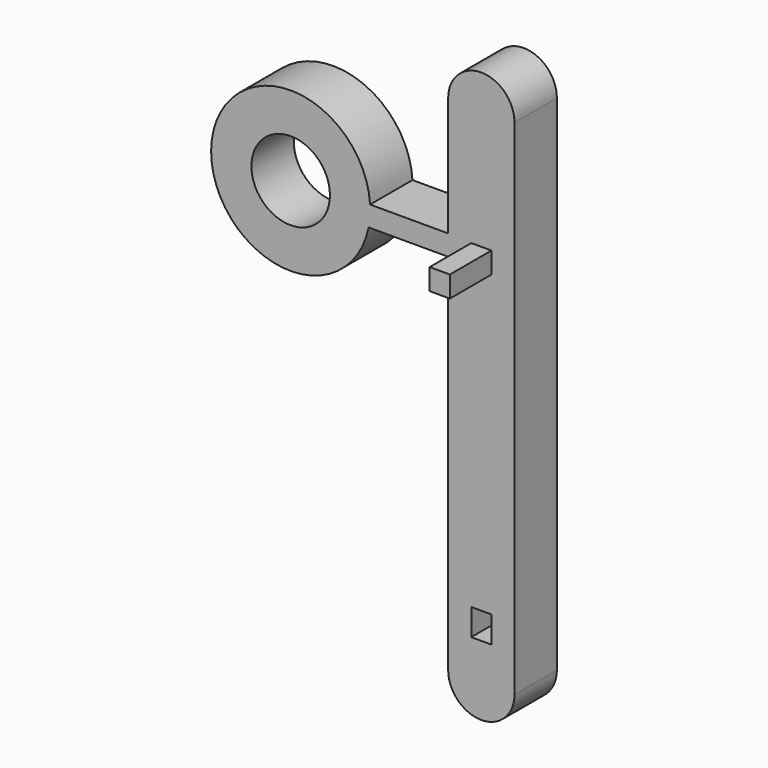
from build123d import *

# Parameters (mm, degrees)
F0_R     = 4.7018325436
F0_W     = 2.4090255611
F0_H     = 3.1813085079
F0_W_2   = 2.413
F0_H_2   = 2.54
F1_DEPTH = 3.175
F2_DEPTH = 9.398
F3_DEPTH = 3.175


# Not quite as in the source:
# - a feature names something its author has since deleted; it is built from what else it names


with BuildPart() as f1:
    # F0 (on Front) → F1 (new body, symmetric)
    with BuildSketch(Plane.XZ):
        with BuildLine():
            ThreePointArc((-13.3044686056, 15.3006398952), (-13.3088027932, 15.5879506834), (-13.3218014117, 15.875))
            ThreePointArc((-13.3218014117, 15.875), (-32.3313565604, 15.9637766028), (-13.49375, 13.4112))
            ThreePointArc((-13.49375, 13.4112), (-13.3519070859, 14.3511912968), (-13.3044686056, 15.3006398952))
        make_face()
        with Locations((-22.8294686056, 15.3006398952)):
            Circle(F0_R, mode=Mode.SUBTRACT)
        with BuildLine():
            Line((-3.96875, 13.4112), (-3.96875, 15.875))
            Line((-3.96875, 15.875), (-13.3218014117, 15.875))
            ThreePointArc((-13.3218014117, 15.875), (-13.3088027932, 15.5879506834), (-13.3044686056, 15.3006398952))
            ThreePointArc((-13.3044686056, 15.3006398952), (-13.3519070859, 14.3511912968), (-13.49375, 13.4112))
            Line((-13.49375, 13.4112), (-3.96875, 13.4112))
        make_face()
        with BuildLine():
            Line((3.96875, -30.1625), (3.96875, 30.1625))
            ThreePointArc((3.96875, 30.1625), (0, 34.13125), (-3.96875, 30.1625))
            Line((-3.96875, 30.1625), (-3.96875, 15.875))
            Line((-3.96875, 15.875), (-3.96875, 13.4112))
            Line((-3.96875, 13.4112), (-3.96875, -30.1625))
            ThreePointArc((-3.96875, -30.1625), (0, -34.13125), (3.96875, -30.1625))
        make_face()
        with Locations((0, -24.1956412792)):
            Rectangle(F0_W, F0_H, mode=Mode.SUBTRACT)
        with Locations((0, 14.4846439362)):
            Rectangle(F0_W_2, F0_H_2, mode=Mode.SUBTRACT)
    extrude(amount=F1_DEPTH, both=True)

    # F0 (on Front) → F2 (join)
    with BuildSketch(Plane.XZ):
        with Locations((0, 14.4846439362)):
            Rectangle(F0_W_2, F0_H_2)
    extrude(amount=F2_DEPTH)

    # F0 (on Front) → F3 (join)
    with BuildSketch(Plane.XZ):
        with Locations((0, 14.4846439362)):
            Rectangle(F0_W_2, F0_H_2)
    extrude(amount=-F3_DEPTH)


solid = f1.part
